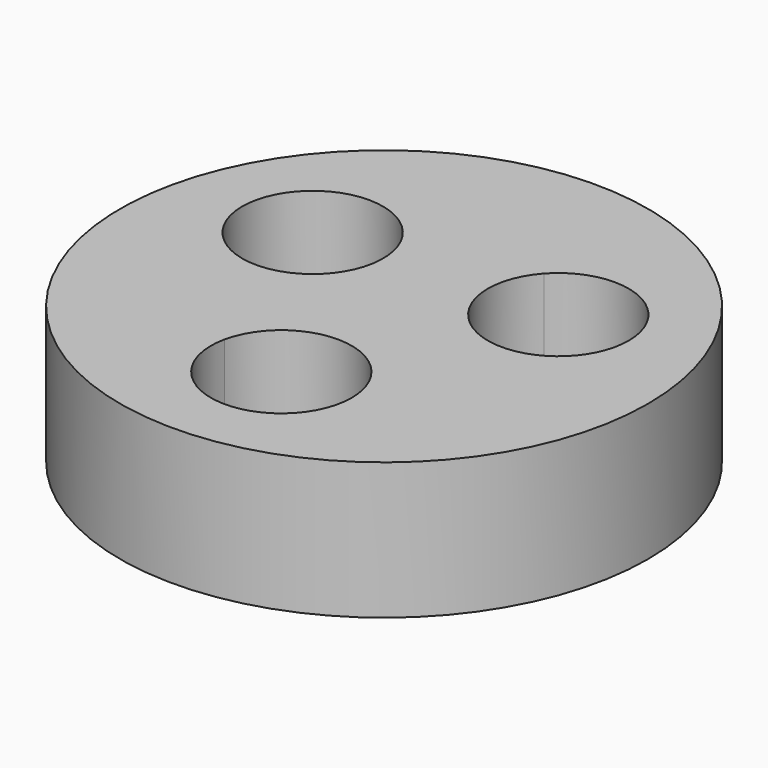
from build123d import *

# Parameters (mm, degrees)
F0_R     = 9.65
F1_DEPTH = 5
F3_DEPTH = 5.001


with BuildPart() as f1:
    # F0 (on Top) → F1 (new body)
    with BuildSketch(Plane.XY):
        Circle(F0_R)
    extrude(amount=F1_DEPTH)

    # F2 (on face) → F3 (cut, through all)
    with BuildSketch(Plane.XY.offset(5)):
        with BuildLine():
            ThreePointArc((2.3027162866, 4.4381863079), (2.0398793124, 1.311303699), (4.9936375982, 0.252157763))
            ThreePointArc((4.9936375982, 0.252157763), (4.2059367266, 2.7037189669), (2.3027162866, 4.4381863079))
        make_face()
        with BuildLine():
            ThreePointArc((2.3027162866, 4.4381863079), (4.2059367266, 2.7037189669), (4.9936375982, 0.252157763))
            ThreePointArc((4.9936375982, 0.252157763), (6.286676348, 1.1867655636), (6.7809367266, 2.7037189669))
            ThreePointArc((6.7809367266, 2.7037189669), (5.1359454274, 5.1049080091), (2.3027162866, 4.4381863079))
        make_face()
        with BuildLine():
            ThreePointArc((2.8135209468, -4.9943075354), (2.783016007, -4.5991241749), (2.692223946, -4.2133039558))
            ThreePointArc((2.692223946, -4.2133039558), (0.2385209468, -4.9943075354), (-2.2784437706, -4.4506958988))
            ThreePointArc((-2.2784437706, -4.4506958988), (-0.0348294261, -7.5547576079), (2.8135209468, -4.9943075354))
        make_face()
        with BuildLine():
            ThreePointArc((-2.2784437706, -4.4506958988), (0.2385209468, -4.9943075354), (2.692223946, -4.2133039558))
            ThreePointArc((2.692223946, -4.2133039558), (0.1156826592, -2.4222391547), (-2.2784437706, -4.4506958988))
        make_face()
        with BuildLine():
            ThreePointArc((-1.8694576733, 2.2905885685), (-2.090367679, 3.3340852377), (-2.7151938276, 4.1985381359))
            ThreePointArc((-2.7151938276, 4.1985381359), (-4.4444576733, 2.2905885685), (-4.9949402326, -0.224882352))
            ThreePointArc((-4.9949402326, -0.224882352), (-2.8299713139, 0.2845828867), (-1.8694576733, 2.2905885685))
        make_face()
        with BuildLine():
            ThreePointArc((-4.9949402326, -0.224882352), (-4.4444576733, 2.2905885685), (-2.7151938276, 4.1985381359))
            ThreePointArc((-2.7151938276, 4.1985381359), (-6.7333533751, 3.4702416812), (-4.9949402326, -0.224882352))
        make_face()
    extrude(amount=-F3_DEPTH, mode=Mode.SUBTRACT)


solid = f1.part
